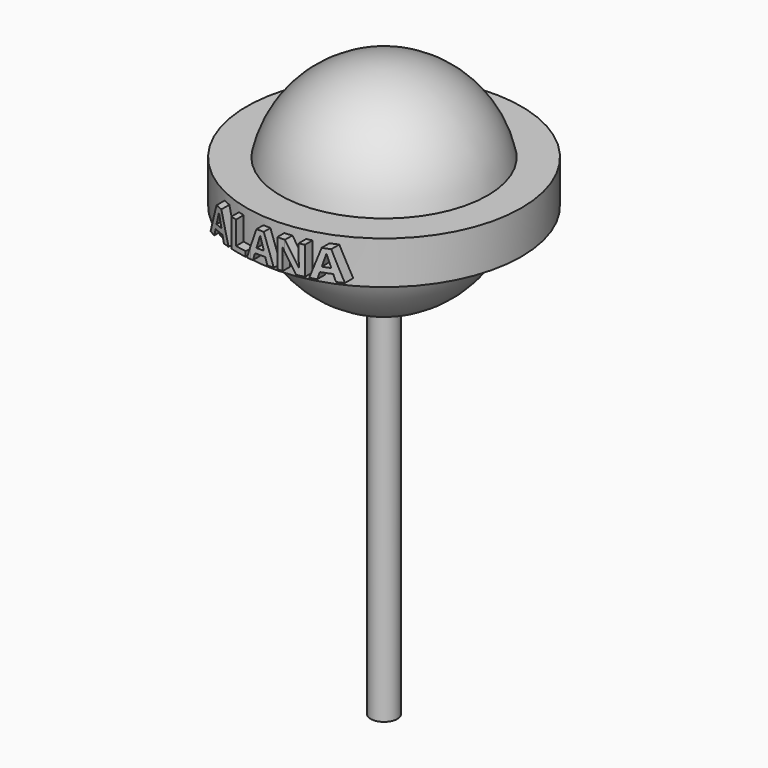
from build123d import *

# Parameters (mm, degrees)
F2_TEXT_SIZE = 6.4102855201
F3_DEPTH     = 23.622


# Not quite as in the source:
# - Text() gives the source's letters only with a copy of the font that has no kerning and outlines rounded to 1/6400 em; it was checked with that copy


with BuildPart() as f1:
    # F0 (on Front) → F1 (revolve)
    with BuildSketch(Plane.XZ):
        with BuildLine():
            Line((0, -13.5924331844), (0, -17.1515149727))
            ThreePointArc((0, -17.1515149727), (1.0833800373, -17.1172647802), (2.1624332294, -17.0146509923))
            Line((2.1624332294, -17.0146509923), (2.1624332294, -13.5924331844))
            Line((2.1624332294, -13.5924331844), (0, -13.5924331844))
        make_face()
        with BuildLine():
            ThreePointArc((2.1624332294, -17.0146509923), (1.0833800373, -17.1172647802), (0, -17.1515149727))
            Line((0, -17.1515149727), (0, -75.9940519929))
            Line((0, -75.9940519929), (2.1624332294, -75.9940519929))
            Line((2.1624332294, -75.9940519929), (2.1624332294, -17.0146509923))
        make_face()
        with BuildLine():
            Line((2.1624332294, -13.5924331844), (2.1624332294, -17.0146509923))
            ThreePointArc((2.1624332294, -17.0146509923), (11.6497974371, -12.5879579573), (16.7965942456, -3.4711507615))
            Line((16.7965942456, -3.4711507615), (2.1624332294, -3.4711507615))
            Line((2.1624332294, -3.4711507615), (2.1624332294, 3.4711507615))
            Line((2.1624332294, 3.4711507615), (16.7965942456, 3.4711507615))
            ThreePointArc((16.7965942456, 3.4711507615), (10.8314119948, 13.2986833957), (0, 17.1515149727))
            Line((0, 17.1515149727), (0, -13.5924331844))
            Line((0, -13.5924331844), (2.1624332294, -13.5924331844))
        make_face()
        with BuildLine():
            Line((2.1624332294, -3.4711507615), (16.7965942456, -3.4711507615))
            ThreePointArc((16.7965942456, -3.4711507615), (17.1515149727, 0), (16.7965942456, 3.4711507615))
            Line((16.7965942456, 3.4711507615), (2.1624332294, 3.4711507615))
            Line((2.1624332294, 3.4711507615), (2.1624332294, -3.4711507615))
        make_face()
        with BuildLine():
            ThreePointArc((16.7965942456, 3.4711507615), (17.1515149727, 0), (16.7965942456, -3.4711507615))
            Line((16.7965942456, -3.4711507615), (22.2810888663, -3.4711507615))
            Line((22.2810888663, -3.4711507615), (22.2810888663, 3.4711507615))
            Line((22.2810888663, 3.4711507615), (16.7965942456, 3.4711507615))
        make_face()
    revolve(axis=Axis((0, 0, 25.3884196281), (0, 0, 1)))

    # F2 (on Front) → F3 (join)
    with BuildSketch(Plane.XZ):
        with Locations((-11.4414086565, -2.3700017482)):
            Text('ALANA', F2_TEXT_SIZE, font='Open Sans', font_style=FontStyle.BOLD, text_align=(TextAlign.LEFT, TextAlign.BOTTOM))
    extrude(amount=F3_DEPTH)

    # F4 (on Front) → F5 (revolve, cut)
    with BuildSketch(Plane.XZ):
        Polygon((23.7810888663, 4.9711507615), (23.7810888663, -4.9711507615), (17.3179358244, -4.9711507615), (23.9894334227, -13.5377270505), (31.9903567433, -11.3247053102), (38.6294238269, -8.8975916281), (38.6294238269, 7.9554195851), (25.1810625196, 24.9786635265), (14.1159519553, 13.0623939782), (16.8014001101, 4.9711507615), align=None)
    revolve(axis=Axis((0, 0, 18.0184356868), (0, 0, 1)), mode=Mode.SUBTRACT)


solid = f1.part
